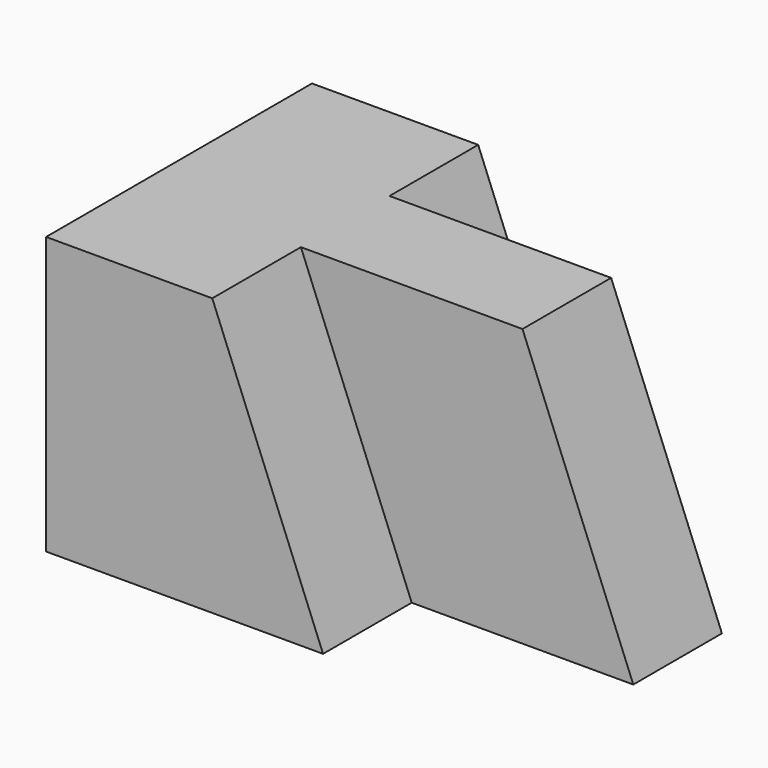
from build123d import *

# Parameters (mm, degrees)
F1_DEPTH = 31.75
F3_DEPTH = 12.7
F5_DEPTH = 12.7
F7_DEPTH = 12.7


# Not quite as in the source:
# - a length typed as a fraction of an inch, garbled in the dataset ("3 / 203.2 mm" for 3/8 in), is restored


with BuildPart() as f1:
    # F0 (on Top) → F1 (new body)
    with BuildSketch(Plane.XY):
        Polygon((31.75, 0), (0, 0), (0, -38.1), (31.75, -38.1), (31.75, -25.4), (57.15, -25.4), (57.15, -12.7), (31.75, -12.7), align=None)
    extrude(amount=F1_DEPTH)

    # F2 (on face) → F3 (cut)
    with BuildSketch(Plane.XZ.offset(38.1)):
        Polygon((19.05, 31.75), (31.75, 0), (31.75, 31.75), align=None)
    extrude(amount=-F3_DEPTH, mode=Mode.SUBTRACT)

    # F4 (on face) → F5 (cut)
    with BuildSketch(Plane.XZ.offset(25.4)):
        Polygon((44.45, 31.75), (57.15, 0), (57.15, 31.75), align=None)
    extrude(amount=-F5_DEPTH, mode=Mode.SUBTRACT)

    # F6 (on face) → F7 (cut)
    with BuildSketch(Plane(origin=(0, 0, 0), x_dir=(-1, 0, 0), z_dir=(0, 1, 0))):
        Polygon((-31.75, 31.75), (-31.75, 0), (-19.05, 31.75), align=None)
    extrude(amount=-F7_DEPTH, mode=Mode.SUBTRACT)


solid = f1.part
